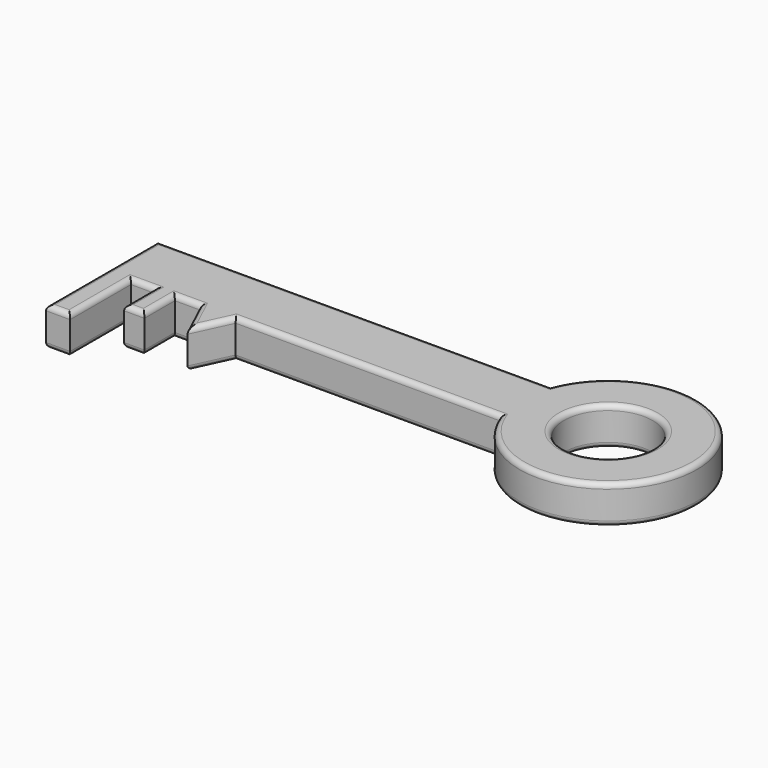
from build123d import *

# Parameters (mm, degrees)
F0_W     = 9.4753347638
F0_H     = 30
F0_R     = 17.5
F1_DEPTH = 15
F2_R     = 2
F3_R     = 2


# Not quite as in the source:
# - a feature names something its author has since deleted; it is built from what else it names


with BuildPart() as f1:
    # F0 (on Top) → F1 (new body)
    with BuildSketch(Plane.XY):
        with Locations((-149.2113988997, 5.7397255301)):
            Rectangle(F0_W, F0_H)
        Polygon((1.0509337184, 20.7397255301), (1.0509337184, 45.7397255301), (-153.9490662816, 45.7397255301), (-153.9490662816, 20.7397255301), (-144.4737315178, 20.7397255301), (-135.1745359898, 20.7397255301), (-134.4737315178, 20.7397255301), (-127.1745359898, 20.7397255301), (-117.1745359898, 20.7397255301), (-103.1745359898, 20.7397255301), align=None)
        with BuildLine():
            ThreePointArc((1.0509337184, 20.7397255301), (68.742675795, 33.2397255301), (1.0509337184, 45.7397255301))
            Line((1.0509337184, 45.7397255301), (1.0509337184, 20.7397255301))
        make_face()
        with Locations((33.742675795, 33.2397255301)):
            Circle(F0_R, mode=Mode.SUBTRACT)
        Polygon((-134.4737315178, 20.7397255301), (-135.1745359898, 20.7397255301), (-135.1745359898, 5.7397255301), (-134.4737315178, 5.7397255301), (-127.1745359898, 5.7397255301), (-127.1745359898, 20.7397255301), align=None)
        Polygon((-110.1745359898, 5.7397255301), (-103.1745359898, 20.7397255301), (-117.1745359898, 20.7397255301), align=None)
    extrude(amount=F1_DEPTH)

    # F2
    f2_edges = [f1.edges().sort_by_distance(p)[0] for p in [
        (68.742676, 33.239726, 0),
        (16.242676, 33.239726, 0),
        (-51.061801, 20.739726, 0),
        (-106.674536, 13.239726, 0),
        (-127.174536, 13.239726, 0),
        (-122.174536, 20.739726, 0),
        (-113.674536, 13.239726, 0),
        (-135.174536, 13.239726, 0),
        (-131.174536, 5.739726, 0),
        (-139.824134, 20.739726, 0),
        (-144.473732, 5.739726, 0),
        (-149.211399, -9.260274, 0),
        (-153.949066, 18.239726, 0),
    ]]
    fillet(f2_edges, radius=F2_R)

    # F3
    f3_edges = [f1.edges().sort_by_distance(p)[0] for p in [
        (-149.211399, -9.260274, 15),
        (-144.473732, 5.739726, 15),
        (-139.824134, 20.739726, 15),
        (-135.174536, 13.239726, 15),
        (-131.174536, 5.739726, 15),
        (-127.174536, 13.239726, 15),
        (-122.174536, 20.739726, 15),
        (-113.674536, 13.239726, 15),
        (-106.674536, 13.239726, 15),
        (-51.061801, 20.739726, 15),
        (68.742676, 33.239726, 15),
        (-76.449066, 45.739726, 15),
        (-153.949066, 18.239726, 15),
        (16.242676, 33.239726, 15),
    ]]
    fillet(f3_edges, radius=F3_R)


solid = f1.part
